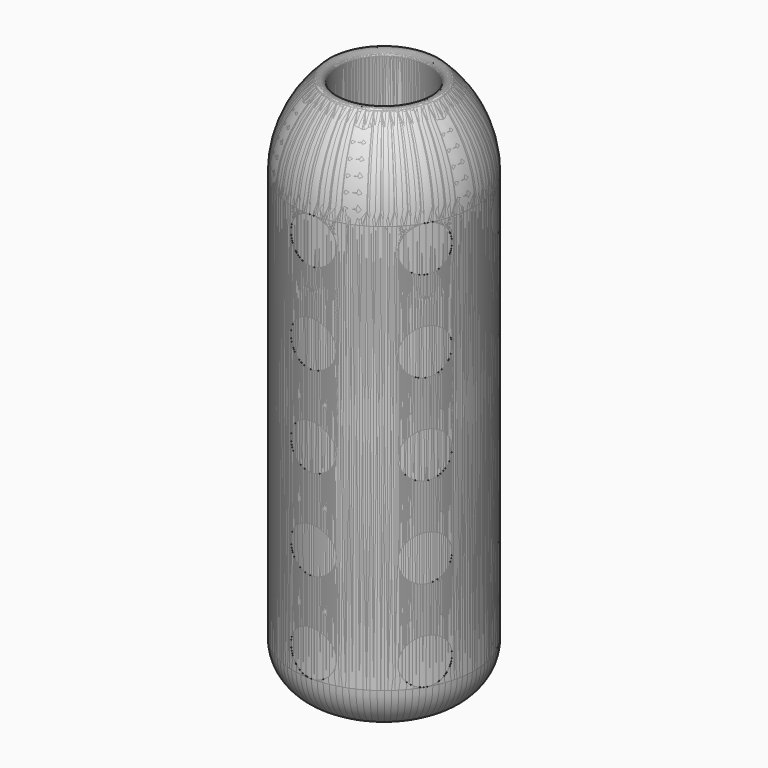
from build123d import *

# Parameters (mm, degrees)
F2_R          = 12.7
F3_DEPTH      = 152.4
F4_R          = 1.524
F5_R          = 12.69999
F6_R          = 6.35
F7_DEPTH      = 25.4010001
F7_DEPTH_BACK = 25.4010001
F9_COUNT      = 6


# Not quite as in the source:
# - a fillet or chamfer is up to 0.001 mm smaller than in the source, because OpenCascade refuses the exact size


with BuildPart() as f1:
    # F0 (on Front) → F1 (revolve)
    with BuildSketch(Plane.XZ):
        with BuildLine():
            Line((0, 152.4), (0, 0))
            Line((0, 0), (25.4, 0))
            Line((25.4, 0), (25.4, 127))
            ThreePointArc((25.4, 127), (22.0480633142, 141.1990316571), (12.7, 152.4))
            Line((12.7, 152.4), (0, 152.4))
        make_face()
    revolve(axis=Axis((0, 0, 76.2), (0, 0, 1)))

    # F2 (on Top) → F3 (cut)
    with BuildSketch(Plane.XY):
        Circle(F2_R)
    extrude(amount=F3_DEPTH, mode=Mode.SUBTRACT)

    # F4
    f4_edges = [f1.edges().sort_by_distance(p)[0] for p in [
        (-12.7, 0, 152.4),
    ]]
    fillet(f4_edges, radius=F4_R)

    # F5 (radius 12.7 in the source; OpenCascade refuses exactly that, so slightly less here)
    f5_edges = [f1.edges().sort_by_distance(p)[0] for p in [
        (-25.4, 0, 0),
    ]]
    fillet(f5_edges, radius=F5_R)

    # F6 (on Front) → F7 (cut, two sides)
    with BuildSketch(Plane.XZ) as f7_sk:
        with Locations((0, 19.05)):
            Circle(F6_R)
        with Locations((0, 44.45)):
            Circle(F6_R)
        with Locations((0, 69.8500026468)):
            Circle(F6_R)
        with Locations((0, 95.2500026468)):
            Circle(F6_R)
        with Locations((0, 120.6500026468)):
            Circle(F6_R)
    extrude(amount=-F7_DEPTH, mode=Mode.SUBTRACT)
    extrude(f7_sk.sketch, amount=F7_DEPTH_BACK, mode=Mode.SUBTRACT)


with BuildPart() as f9_1:
    # F9: instance of F1
    add(f1.part.rotate(Axis((0, 0, 76.2), (0, 0, 1)), 1 * 360 / F9_COUNT))


with BuildPart() as f9_2:
    # F9: instance of F1
    add(f1.part.rotate(Axis((0, 0, 76.2), (0, 0, 1)), 2 * 360 / F9_COUNT))


with BuildPart() as f9_3:
    # F9: instance of F1
    add(f1.part.rotate(Axis((0, 0, 76.2), (0, 0, 1)), 3 * 360 / F9_COUNT))


with BuildPart() as f9_4:
    # F9: instance of F1
    add(f1.part.rotate(Axis((0, 0, 76.2), (0, 0, 1)), 4 * 360 / F9_COUNT))


with BuildPart() as f9_5:
    # F9: instance of F1
    add(f1.part.rotate(Axis((0, 0, 76.2), (0, 0, 1)), 5 * 360 / F9_COUNT))


solid = Compound([f1.part, f9_1.part, f9_2.part, f9_3.part, f9_4.part, f9_5.part])
